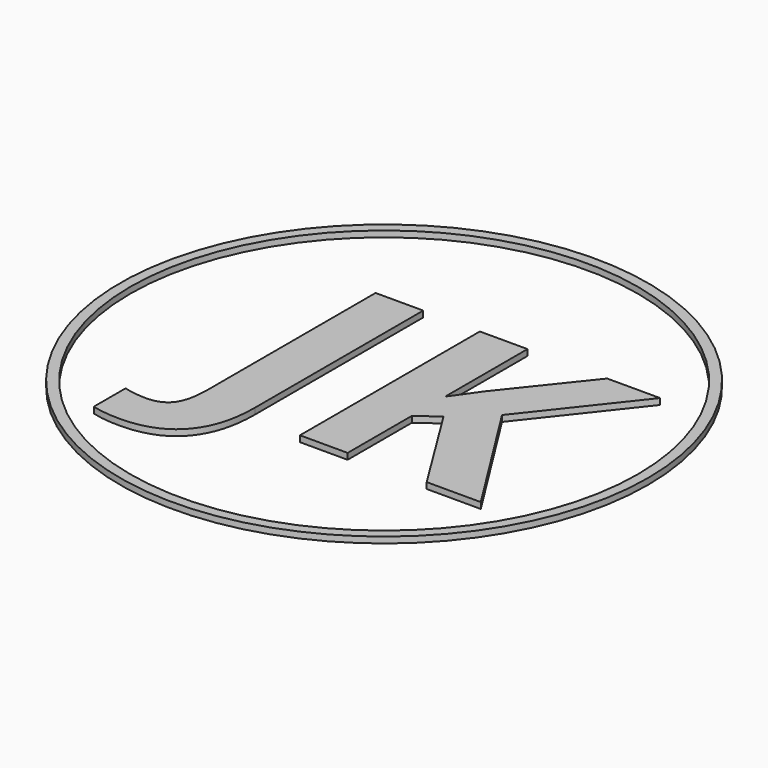
from build123d import *

# Parameters (mm, degrees)
F1_TEXT_SIZE = 19.6993015272
F2_R         = 16.51
F2_R_2       = 15.875
F3_DEPTH     = 0.381


# Not quite as in the source:
# - Text() gives the source's letters only with a copy of the font that has no kerning and outlines rounded to 1/6400 em; it was checked with that copy


with BuildPart() as f3:
    # F1 (on offset) + F2 (on offset) → F3 (new body)
    with BuildSketch(Plane.XY.offset(3.302)):
        with Locations((-7.8812596188, -7.0917485498)):
            Text('JK', F1_TEXT_SIZE, font='Open Sans', font_style=FontStyle.BOLD, text_align=(TextAlign.LEFT, TextAlign.BOTTOM))
    with BuildSketch(Plane.XY.offset(3.302)):
        Circle(F2_R)
        Circle(F2_R_2, mode=Mode.SUBTRACT)
    extrude(amount=-F3_DEPTH)


solid = f3.part
